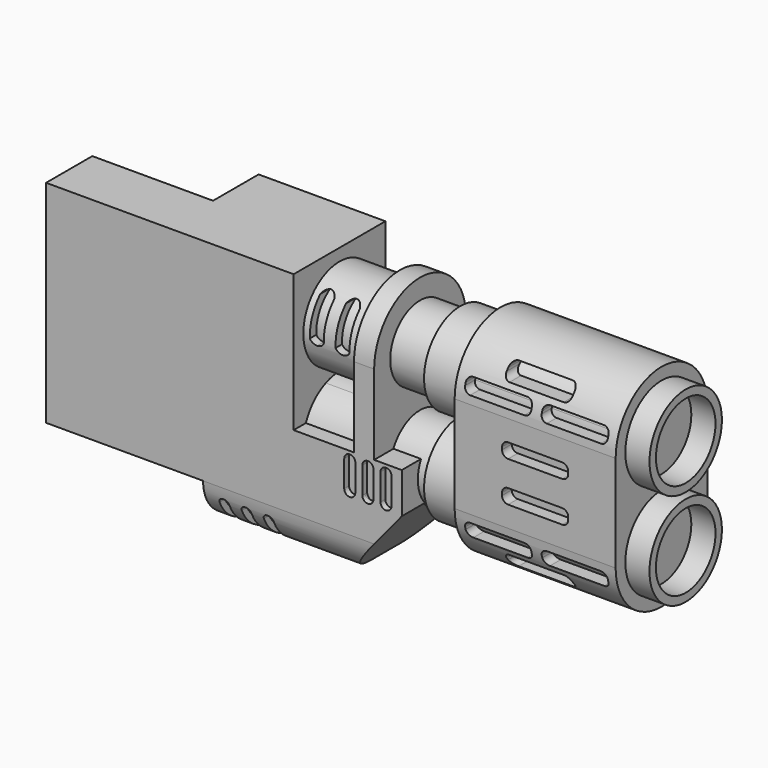
from build123d import *

# Parameters (mm, degrees)
F1_DEPTH  = 5.7
F0_W      = 6
F0_H      = 5.25
F2_DEPTH  = 2.87
F3_R      = 1.85
F4_DEPTH  = 3
F6_DEPTH  = 1
F7_R      = 1.85
F8_DEPTH  = 2
F9_R      = 2.25
F9_R_2    = 1.85
F10_DEPTH = 2
F11_R     = 2.25
F12_DEPTH = 8
F13_R     = 2.25
F13_R_2   = 1.85
F14_DEPTH = 1.2
F15_W     = 0.3467793576
F15_H     = 1.6864892095
F16_DEPTH = 6
F17_DEPTH = 6
F18_DEPTH = 5
F20_DEPTH = 8
F22_DEPTH = 7.25
F24_DEPTH = 5.7
F26_DEPTH = 8.5
F27_DEPTH = 6
F28_DEPTH = 25
F30_DEPTH = 5


with BuildPart() as f1:
    # F0 (on Front) → F1 (new body)
    with BuildSketch(Plane.XZ):
        Polygon((-20.4995705068, 5.25), (-20.4995705068, 0), (-8.1995705068, 0), (-8.1995705068, 10.5), (-14.4995705068, 10.5), (-14.4995705068, 5.25), align=None)
    extrude(amount=-F1_DEPTH)

    # F0 (on Front) → F2 (join)
    with BuildSketch(Plane.XZ):
        with Locations((-17.4995705068, 7.875)):
            Rectangle(F0_W, F0_H)
    extrude(amount=-F2_DEPTH)

    # F3 (on face) → F4 (join)
    with BuildSketch(Plane.YZ.offset(-8.1995705068)):
        with BuildLine():
            ThreePointArc((1.9950740164, 5.56875), (2.85, 5.7), (3.7049259836, 5.56875))
            ThreePointArc((3.7049259836, 5.56875), (4.7189680927, 6.3972197845), (5.1, 7.65))
            ThreePointArc((5.1, 7.65), (1.5972197845, 9.5189680927), (1.9950740164, 5.56875))
        make_face()
        with Locations((2.85, 7.65)):
            Circle(F3_R, mode=Mode.SUBTRACT)
        with Locations((2.85, 7.65)):
            Circle(F3_R)
        with BuildLine():
            ThreePointArc((5.1, 2.85), (4.7189680927, 4.1027802155), (3.7049259836, 4.93125))
            ThreePointArc((3.7049259836, 4.93125), (2.85, 4.8), (1.9950740164, 4.93125))
            ThreePointArc((1.9950740164, 4.93125), (1.5972197845, 0.9810319073), (5.1, 2.85))
        make_face()
        with Locations((2.85, 2.85)):
            Circle(F3_R, mode=Mode.SUBTRACT)
        with Locations((2.85, 2.85)):
            Circle(F3_R)
        with BuildLine():
            ThreePointArc((1.9950740164, 4.93125), (2.85, 4.8), (3.7049259836, 4.93125))
            ThreePointArc((3.7049259836, 4.93125), (2.85, 5.1), (1.9950740164, 4.93125))
        make_face()
        with BuildLine():
            ThreePointArc((1.9950740164, 5.56875), (2.85, 5.4), (3.7049259836, 5.56875))
            ThreePointArc((3.7049259836, 5.56875), (2.85, 5.7), (1.9950740164, 5.56875))
        make_face()
    extrude(amount=F4_DEPTH)

    # F5 (on face) → F6 (join)
    with BuildSketch(Plane.YZ.offset(-5.1995705068)):
        with BuildLine():
            Line((5.7, 2.85), (5.7, 7.65))
            ThreePointArc((5.7, 7.65), (2.85, 10.5), (0, 7.65))
            Line((0, 7.65), (0, 2.85))
            ThreePointArc((0, 2.85), (2.85, 0), (5.7, 2.85))
        make_face()
    extrude(amount=F6_DEPTH)

    # F7 (on face) → F8 (join)
    with BuildSketch(Plane.YZ.offset(-4.1995705068)):
        with Locations((2.85, 7.65)):
            Circle(F7_R)
        with Locations((2.85, 2.85)):
            Circle(F7_R)
    extrude(amount=F8_DEPTH)

    # F9 (on face) → F10 (join)
    with BuildSketch(Plane.YZ.offset(-2.1995705068)):
        with Locations((2.85, 7.65)):
            Circle(F9_R)
        with Locations((2.85, 7.65)):
            Circle(F9_R_2, mode=Mode.SUBTRACT)
        with Locations((2.85, 7.65)):
            Circle(F9_R_2)
        with Locations((2.85, 2.85)):
            Circle(F9_R)
    extrude(amount=F10_DEPTH)

    # F11 (on face) → F12 (join)
    with BuildSketch(Plane.YZ.offset(-0.1995705068)):
        with BuildLine():
            ThreePointArc((5.7, 7.65), (2.85, 10.5), (0, 7.65))
            Line((0, 7.65), (0, 2.85))
            ThreePointArc((0, 2.85), (2.85, 0), (5.7, 2.85))
            Line((5.7, 2.85), (5.7, 7.65))
        make_face()
        with Locations((2.85, 7.65)):
            Circle(F11_R, mode=Mode.SUBTRACT)
        with Locations((2.85, 7.65)):
            Circle(F11_R)
    extrude(amount=F12_DEPTH)

    # F13 (on face) → F14 (join)
    with BuildSketch(Plane.YZ.offset(7.8004294932)):
        with Locations((2.85, 7.65)):
            Circle(F13_R)
        with Locations((2.85, 7.65)):
            Circle(F13_R_2, mode=Mode.SUBTRACT)
        with Locations((2.85, 2.85)):
            Circle(F13_R)
        with Locations((2.85, 2.85)):
            Circle(F13_R_2, mode=Mode.SUBTRACT)
    extrude(amount=F14_DEPTH)

    # F15 (on face) → F16 (cut)
    with BuildSketch(Plane.XZ):
        with BuildLine():
            Line((-7.5294733979, 9.2348763719), (-7.5294733979, 9.4476234936))
            ThreePointArc((-7.5294733979, 9.4476234936), (-7.7328924608, 9.3901980476), (-7.8762527555, 9.2348763719))
            Line((-7.8762527555, 9.2348763719), (-7.5294733979, 9.2348763719))
        make_face()
        with BuildLine():
            ThreePointArc((-7.1826940402, 9.2348763719), (-7.3260543349, 9.3901980476), (-7.5294733979, 9.4476234936))
            Line((-7.5294733979, 9.4476234936), (-7.5294733979, 9.2348763719))
            Line((-7.5294733979, 9.2348763719), (-7.1826940402, 9.2348763719))
        make_face()
        with Locations((-7.3560837191, 8.3916317672)):
            Rectangle(F15_W, F15_H)
        with Locations((-7.7028630767, 8.3916317672)):
            Rectangle(F15_W, F15_H)
        with BuildLine():
            Line((-7.5294733979, 7.3356400407), (-7.5294733979, 7.5483871624))
            Line((-7.5294733979, 7.5483871624), (-7.8762527555, 7.5483871624))
            ThreePointArc((-7.8762527555, 7.5483871624), (-7.7328924608, 7.3930654867), (-7.5294733979, 7.3356400407))
        make_face()
        with BuildLine():
            Line((-7.1826940402, 7.5483871624), (-7.5294733979, 7.5483871624))
            Line((-7.5294733979, 7.5483871624), (-7.5294733979, 7.3356400407))
            ThreePointArc((-7.5294733979, 7.3356400407), (-7.3260543349, 7.3930654867), (-7.1826940402, 7.5483871624))
        make_face()
    extrude(amount=-F16_DEPTH, mode=Mode.SUBTRACT)

    # F15 (on face) → F17 (cut)
    with BuildSketch(Plane.XZ):
        with BuildLine():
            ThreePointArc((-5.9049502015, 9.2348763719), (-6.2517295592, 9.4476234936), (-6.5985089168, 9.2348763719))
            Line((-6.5985089168, 9.2348763719), (-6.5985089168, 7.5483871624))
            ThreePointArc((-6.5985089168, 7.5483871624), (-6.2517295592, 7.3356400407), (-5.9049502015, 7.5483871624))
            Line((-5.9049502015, 7.5483871624), (-5.9049502015, 9.2348763719))
        make_face()
    extrude(amount=-F17_DEPTH, mode=Mode.SUBTRACT)

    # F3 (on face) → F18 (join)
    with BuildSketch(Plane.YZ.offset(-8.1995705068)):
        with Locations((2.85, 7.65)):
            Circle(F3_R)
    extrude(amount=F18_DEPTH)

    # F19 (on face) → F20 (cut)
    with BuildSketch(Plane.XZ):
        with BuildLine():
            Line((0.5530155201, 8.0402910583), (3.2419295742, 8.0402910583))
            ThreePointArc((3.2419295742, 8.0402910583), (3.4540616085, 8.1281590239), (3.5419295742, 8.3402910583))
            Line((3.5419295742, 8.3402910583), (3.5419295742, 8.4660525121))
            ThreePointArc((3.5419295742, 8.4660525121), (3.4540616085, 8.6781845464), (3.2419295742, 8.7660525121))
            Line((3.2419295742, 8.7660525121), (0.5530155201, 8.7660525121))
            ThreePointArc((0.5530155201, 8.7660525121), (0.3408834857, 8.6781845464), (0.2530155201, 8.4660525121))
            Line((0.2530155201, 8.4660525121), (0.2530155201, 8.3402910583))
            ThreePointArc((0.2530155201, 8.3402910583), (0.3408834857, 8.1281590239), (0.5530155201, 8.0402910583))
        make_face()
        with BuildLine():
            Line((2.2455907629, 9.0279276721), (4.9345048171, 9.0279276721))
            ThreePointArc((4.9345048171, 9.0279276721), (5.1466368514, 9.1157956378), (5.2345048171, 9.3279276721))
            Line((5.2345048171, 9.3279276721), (5.2345048171, 9.4536891259))
            ThreePointArc((5.2345048171, 9.4536891259), (5.1466368514, 9.6658211603), (4.9345048171, 9.7536891259))
            Line((4.9345048171, 9.7536891259), (2.2455907629, 9.7536891259))
            ThreePointArc((2.2455907629, 9.7536891259), (2.0334587286, 9.6658211603), (1.9455907629, 9.4536891259))
            Line((1.9455907629, 9.4536891259), (1.9455907629, 9.3279276721))
            ThreePointArc((1.9455907629, 9.3279276721), (2.0334587286, 9.1157956378), (2.2455907629, 9.0279276721))
        make_face()
        with BuildLine():
            Line((4.0589294122, 8.4660525121), (4.0589294122, 8.3402910583))
            ThreePointArc((4.0589294122, 8.3402910583), (4.1467973779, 8.1281590239), (4.3589294122, 8.0402910583))
            Line((4.3589294122, 8.0402910583), (7.0478434663, 8.0402910583))
            ThreePointArc((7.0478434663, 8.0402910583), (7.2599755007, 8.1281590239), (7.3478434663, 8.3402910583))
            Line((7.3478434663, 8.3402910583), (7.3478434663, 8.4660525121))
            ThreePointArc((7.3478434663, 8.4660525121), (7.2599755007, 8.6781845464), (7.0478434663, 8.7660525121))
            Line((7.0478434663, 8.7660525121), (4.3589294122, 8.7660525121))
            ThreePointArc((4.3589294122, 8.7660525121), (4.1467973779, 8.6781845464), (4.0589294122, 8.4660525121))
        make_face()
        with BuildLine():
            Line((2.4559724661, 5.8871259913), (5.1448865202, 5.8871259913))
            ThreePointArc((5.1448865202, 5.8871259913), (5.3570185546, 5.9749939569), (5.4448865202, 6.1871259913))
            Line((5.4448865202, 6.1871259913), (5.4448865202, 6.3128740087))
            ThreePointArc((5.4448865202, 6.3128740087), (5.3570185546, 6.5250060431), (5.1448865202, 6.6128740087))
            Line((5.1448865202, 6.6128740087), (2.4559724661, 6.6128740087))
            ThreePointArc((2.4559724661, 6.6128740087), (2.2438404318, 6.5250060431), (2.1559724661, 6.3128740087))
            Line((2.1559724661, 6.3128740087), (2.1559724661, 6.1871259913))
            ThreePointArc((2.1559724661, 6.1871259913), (2.2438404318, 5.9749939569), (2.4559724661, 5.8871259913))
        make_face()
        with BuildLine():
            Line((5.4448865202, 4.1871259913), (5.4448865202, 4.3128740087))
            ThreePointArc((5.4448865202, 4.3128740087), (5.3570185546, 4.5250060431), (5.1448865202, 4.6128740087))
            Line((5.1448865202, 4.6128740087), (2.4559724661, 4.6128740087))
            ThreePointArc((2.4559724661, 4.6128740087), (2.2438404318, 4.5250060431), (2.1559724661, 4.3128740087))
            Line((2.1559724661, 4.3128740087), (2.1559724661, 4.1871259913))
            ThreePointArc((2.1559724661, 4.1871259913), (2.2438404318, 3.9749939569), (2.4559724661, 3.8871259913))
            Line((2.4559724661, 3.8871259913), (5.1448865202, 3.8871259913))
            ThreePointArc((5.1448865202, 3.8871259913), (5.3570185546, 3.9749939569), (5.4448865202, 4.1871259913))
        make_face()
        with BuildLine():
            Line((7.3478434663, 2.0339474879), (7.3478434663, 2.1597089417))
            ThreePointArc((7.3478434663, 2.1597089417), (7.2599755007, 2.3718409761), (7.0478434663, 2.4597089417))
            Line((7.0478434663, 2.4597089417), (4.3589294122, 2.4597089417))
            ThreePointArc((4.3589294122, 2.4597089417), (4.1467973779, 2.3718409761), (4.0589294122, 2.1597089417))
            Line((4.0589294122, 2.1597089417), (4.0589294122, 2.0339474879))
            ThreePointArc((4.0589294122, 2.0339474879), (4.1467973779, 1.8218154536), (4.3589294122, 1.7339474879))
            Line((4.3589294122, 1.7339474879), (7.0478434663, 1.7339474879))
            ThreePointArc((7.0478434663, 1.7339474879), (7.2599755007, 1.8218154536), (7.3478434663, 2.0339474879))
        make_face()
        with BuildLine():
            ThreePointArc((2.2455907629, 1.4720723279), (2.0334587286, 1.3842043622), (1.9455907629, 1.1720723279))
            Line((1.9455907629, 1.1720723279), (1.9455907629, 1.0463108741))
            ThreePointArc((1.9455907629, 1.0463108741), (2.0334587286, 0.8341788397), (2.2455907629, 0.7463108741))
            Line((2.2455907629, 0.7463108741), (4.9345048171, 0.7463108741))
            ThreePointArc((4.9345048171, 0.7463108741), (5.1466368514, 0.8341788397), (5.2345048171, 1.0463108741))
            Line((5.2345048171, 1.0463108741), (5.2345048171, 1.1720723279))
            ThreePointArc((5.2345048171, 1.1720723279), (5.1466368514, 1.3842043622), (4.9345048171, 1.4720723279))
            Line((4.9345048171, 1.4720723279), (2.2455907629, 1.4720723279))
        make_face()
        with BuildLine():
            Line((3.5419295742, 2.0339474879), (3.5419295742, 2.1597089417))
            ThreePointArc((3.5419295742, 2.1597089417), (3.4540616085, 2.3718409761), (3.2419295742, 2.4597089417))
            Line((3.2419295742, 2.4597089417), (0.5530155201, 2.4597089417))
            ThreePointArc((0.5530155201, 2.4597089417), (0.3408834857, 2.3718409761), (0.2530155201, 2.1597089417))
            Line((0.2530155201, 2.1597089417), (0.2530155201, 2.0339474879))
            ThreePointArc((0.2530155201, 2.0339474879), (0.3408834857, 1.8218154536), (0.5530155201, 1.7339474879))
            Line((0.5530155201, 1.7339474879), (3.2419295742, 1.7339474879))
            ThreePointArc((3.2419295742, 1.7339474879), (3.4540616085, 1.8218154536), (3.5419295742, 2.0339474879))
        make_face()
    extrude(amount=-F20_DEPTH, mode=Mode.SUBTRACT)

    # F21 (on face) → F22 (join)
    with BuildSketch(Plane.YZ.offset(0.2530155201)):
        with BuildLine():
            ThreePointArc((0.7085056024, 8.3402910583), (0.6272919226, 7.9993834609), (0.6, 7.65))
            ThreePointArc((0.6, 7.65), (2.85, 5.4), (5.1, 7.65))
            ThreePointArc((5.1, 7.65), (5.0727080774, 7.9993834609), (4.9914943976, 8.3402910583))
            Line((4.9914943976, 8.3402910583), (0.7085056024, 8.3402910583))
        make_face()
        with BuildLine():
            ThreePointArc((5.1, 7.65), (2.85, 5.4), (0.6, 7.65))
            Line((0.6, 7.65), (0.6, 2.85))
            ThreePointArc((0.6, 2.85), (2.85, 5.1), (5.1, 2.85))
            Line((5.1, 2.85), (5.1, 7.65))
        make_face()
        with BuildLine():
            ThreePointArc((0.7532028478, 8.4660525121), (0.7299215106, 8.4035032839), (0.7085056024, 8.3402910583))
            Line((0.7085056024, 8.3402910583), (4.9914943976, 8.3402910583))
            ThreePointArc((4.9914943976, 8.3402910583), (4.9700784894, 8.4035032839), (4.9467971522, 8.4660525121))
            Line((4.9467971522, 8.4660525121), (0.7532028478, 8.4660525121))
        make_face()
        with BuildLine():
            ThreePointArc((5.1, 2.85), (2.85, 5.1), (0.6, 2.85))
            ThreePointArc((0.6, 2.85), (2.85, 0.6), (5.1, 2.85))
        make_face()
        with BuildLine():
            ThreePointArc((4.9467971522, 8.4660525121), (2.85, 9.9), (0.7532028478, 8.4660525121))
            Line((0.7532028478, 8.4660525121), (4.9467971522, 8.4660525121))
        make_face()
    extrude(amount=F22_DEPTH)

    # F23 (on face) → F24 (join)
    with BuildSketch(Plane.XZ):
        with BuildLine():
            Line((-2.8273389078, 3.6809362173), (-4.1995705068, 3.6809362173))
            Line((-4.1995705068, 3.6809362173), (-5.1995705068, 3.6809362173))
            Line((-5.1995705068, 3.6809362173), (-8.1995705068, 3.6809362173))
            Line((-8.1995705068, 3.6809362173), (-8.1995705068, 0))
            Line((-8.1995705068, 0), (-12.6995705068, 0))
            Line((-12.6995705068, 0), (-12.6995705068, -1.9993729426))
            Line((-12.6995705068, -1.9993729426), (-11.9995705068, -1.9993729426))
            Line((-11.9995705068, -1.9993729426), (-11.9995705068, -0.7709459751))
            ThreePointArc((-11.9995705068, -0.7709459751), (-11.7495705068, -0.5209459751), (-11.4995705068, -0.7709459751))
            Line((-11.4995705068, -0.7709459751), (-11.4995705068, -1.9993729426))
            Line((-11.4995705068, -1.9993729426), (-10.8995705068, -1.9993729426))
            Line((-10.8995705068, -1.9993729426), (-10.8995705068, -0.7709459751))
            ThreePointArc((-10.8995705068, -0.7709459751), (-10.6495705068, -0.5209459751), (-10.3995705068, -0.7709459751))
            Line((-10.3995705068, -0.7709459751), (-10.3995705068, -1.9993729426))
            Line((-10.3995705068, -1.9993729426), (-9.7995705068, -1.9993729426))
            Line((-9.7995705068, -1.9993729426), (-9.7995705068, -0.7709459751))
            ThreePointArc((-9.7995705068, -0.7709459751), (-9.5495705068, -0.5209459751), (-9.2995705068, -0.7709459751))
            Line((-9.2995705068, -0.7709459751), (-9.2995705068, -1.9993729426))
            Line((-9.2995705068, -1.9993729426), (-5.851307267, -1.9993729426))
            Line((-5.851307267, -1.9993729426), (-2.8273389078, 1.6610411514))
            Line((-2.8273389078, 1.6610411514), (-2.8273389078, 3.6809362173))
        make_face()
        with BuildLine():
            ThreePointArc((-5.6852754695, 3.2557594823), (-5.5044114196, 3.5142693523), (-5.1995705068, 3.4329602182))
            ThreePointArc((-5.1995705068, 3.4329602182), (-5.1515888645, 3.3500721674), (-5.1349219995, 3.2557594823))
            Line((-5.1349219995, 3.2557594823), (-5.1349219995, 1.9362178864))
            ThreePointArc((-5.1349219995, 1.9362178864), (-5.4100987345, 1.6610411514), (-5.6852754695, 1.9362178864))
            Line((-5.6852754695, 1.9362178864), (-5.6852754695, 3.2557594823))
        make_face(mode=Mode.SUBTRACT)
        with BuildLine():
            ThreePointArc((-4.7852754695, 3.2557594823), (-4.5100987345, 3.5309362173), (-4.2349219995, 3.2557594823))
            Line((-4.2349219995, 3.2557594823), (-4.2349219995, 1.9362178864))
            ThreePointArc((-4.2349219995, 1.9362178864), (-4.5100987345, 1.6610411514), (-4.7852754695, 1.9362178864))
            Line((-4.7852754695, 1.9362178864), (-4.7852754695, 3.2557594823))
        make_face(mode=Mode.SUBTRACT)
        with BuildLine():
            Line((-3.8852754695, 1.9362178864), (-3.8852754695, 3.2557594823))
            ThreePointArc((-3.8852754695, 3.2557594823), (-3.6100987345, 3.5309362173), (-3.3349219995, 3.2557594823))
            Line((-3.3349219995, 3.2557594823), (-3.3349219995, 1.9362178864))
            ThreePointArc((-3.3349219995, 1.9362178864), (-3.6100987345, 1.6610411514), (-3.8852754695, 1.9362178864))
        make_face(mode=Mode.SUBTRACT)
    extrude(amount=-F24_DEPTH)

    # F25 (on face) → F26 (cut)
    with BuildSketch(Plane(origin=(-12.6995705068, 0, 0), x_dir=(0, -1, 0), z_dir=(-1, 0, 0))):
        with BuildLine():
            Line((-5.7, -1.9993729426), (-3.7, -1.9993729426))
            ThreePointArc((-3.7, -1.9993729426), (-5.1139918467, -1.4138081859), (-5.6999999017, 0))
            Line((-5.7, 0), (-5.7, -1.9993729426))
        make_face()
        with BuildLine():
            Line((0, -1.9993729426), (0, 0))
            ThreePointArc((-9.83e-08, 0), (-0.5860081533, -1.4138081859), (-2, -1.9993729426))
            Line((-2, -1.9993729426), (0, -1.9993729426))
        make_face()
    extrude(amount=-F26_DEPTH, mode=Mode.SUBTRACT)

    # F25 (on face) → F27 (join)
    with BuildSketch(Plane(origin=(-12.6995705068, 0, 0), x_dir=(0, -1, 0), z_dir=(-1, 0, 0))):
        with BuildLine():
            ThreePointArc((-2, -1.6993729426), (-0.7981401907, -1.2016761484), (-0.3000001156, 0))
            Line((-0.3000001156, 0), (-5.3999998844, 0))
            ThreePointArc((-5.3999998844, 0), (-4.9018598093, -1.2016761484), (-3.7, -1.6993729426))
            Line((-3.7, -1.6993729426), (-2, -1.6993729426))
        make_face()
    extrude(amount=-F27_DEPTH)

    # F23 (on face) → F28 (cut)
    with BuildSketch(Plane.XZ):
        with BuildLine():
            Line((-4.2349219995, 1.9362178864), (-4.2349219995, 3.2557594823))
            ThreePointArc((-4.2349219995, 3.2557594823), (-4.5100987345, 3.5309362173), (-4.7852754695, 3.2557594823))
            Line((-4.7852754695, 3.2557594823), (-4.7852754695, 1.9362178864))
            ThreePointArc((-4.7852754695, 1.9362178864), (-4.5100987345, 1.6610411514), (-4.2349219995, 1.9362178864))
        make_face()
        with BuildLine():
            ThreePointArc((-5.1349219995, 3.2557594823), (-5.1515888645, 3.3500721674), (-5.1995705068, 3.4329602182))
            ThreePointArc((-5.1995705068, 3.4329602182), (-5.5044114196, 3.5142693523), (-5.6852754695, 3.2557594823))
            Line((-5.6852754695, 3.2557594823), (-5.6852754695, 1.9362178864))
            ThreePointArc((-5.6852754695, 1.9362178864), (-5.4100987345, 1.6610411514), (-5.1349219995, 1.9362178864))
            Line((-5.1349219995, 1.9362178864), (-5.1349219995, 3.2557594823))
        make_face()
        with BuildLine():
            ThreePointArc((-3.3349219995, 3.2557594823), (-3.6100987345, 3.5309362173), (-3.8852754695, 3.2557594823))
            Line((-3.8852754695, 3.2557594823), (-3.8852754695, 1.9362178864))
            ThreePointArc((-3.8852754695, 1.9362178864), (-3.6100987345, 1.6610411514), (-3.3349219995, 1.9362178864))
            Line((-3.3349219995, 1.9362178864), (-3.3349219995, 3.2557594823))
        make_face()
    extrude(amount=-F28_DEPTH, mode=Mode.SUBTRACT)

    # F29 (on face) → F30 (join)
    with BuildSketch(Plane.YZ.offset(-2.8273389078)):
        with BuildLine():
            Line((1.1073763017, 3.6809362173), (0.3, 3.6809362173))
            Line((0.3, 3.6809362173), (0.3, 1.6610411514))
            Line((0.3, 1.6610411514), (1.1073763017, 1.6610411514))
            Line((1.1073763017, 1.6610411514), (1.1073763017, 2.2289020641))
            ThreePointArc((1.1073763017, 2.2289020641), (1, 2.85), (1.1073763017, 3.4710979359))
            Line((1.1073763017, 3.4710979359), (1.1073763017, 3.6809362173))
        make_face()
        Polygon((5.4, 1.6610411514), (5.4, 3.6809362173), (4.5028898944, 3.6809362173), (4.2673485303, 1.6610411514), align=None)
    extrude(amount=-F30_DEPTH)


solid = f1.part
